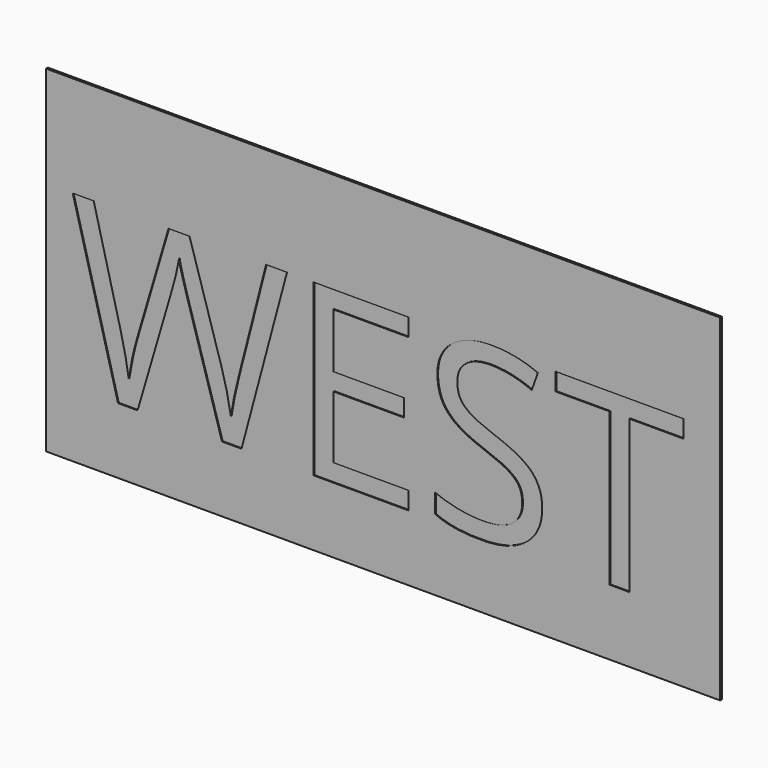
from build123d import *

# Parameters (mm, degrees)
F0_W         = 38.1
F0_H         = 19.05
F1_DEPTH     = 0.127
F2_TEXT_SIZE = 13.472089031
F3_DEPTH     = 0.0508


# Not quite as in the source:
# - Text() gives the source's letters only with a copy of the font that has no kerning and outlines rounded to 1/6400 em; it was checked with that copy


with BuildPart() as f1:
    # F0 (on Front) → F1 (new body)
    with BuildSketch(Plane.XZ):
        with Locations((19.05, 9.525)):
            Rectangle(F0_W, F0_H)
    extrude(amount=F1_DEPTH)

    # F2 (on face) → F3 (cut)
    with BuildSketch(Plane.XZ.offset(0.127)):
        with Locations((1.3300219062, 3.7257757824)):
            Text('WEST', F2_TEXT_SIZE, font='Open Sans', text_align=(TextAlign.LEFT, TextAlign.BOTTOM))
    extrude(amount=-F3_DEPTH, mode=Mode.SUBTRACT)


solid = f1.part
